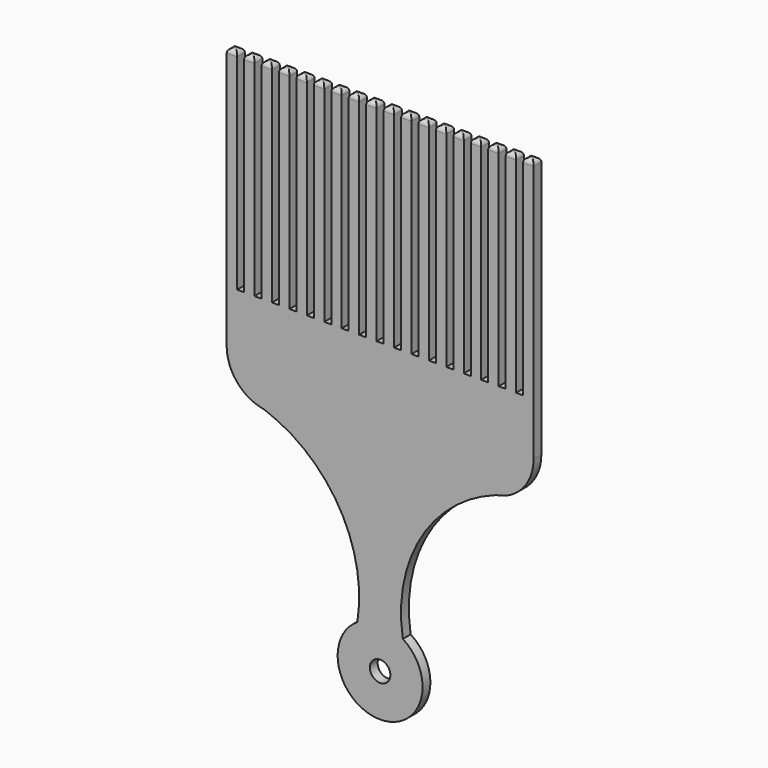
from build123d import *

# Parameters (mm, degrees)
F0_R     = 3.7382012242
F1_DEPTH = 3.556
F3_SCALE = 0.8
F4_R     = 1.27


with BuildPart() as f1:
    # F0 (on Front) → F1 (new body)
    with BuildSketch(Plane.XZ):
        with BuildLine():
            Line((-52.07, 181.6023319495), (-55.88, 181.6023319495))
            Line((-55.88, 181.6023319495), (-55.88, 86.1316665151))
            ThreePointArc((-55.88, 86.1316665151), (-52.0040063032, 75.6508869522), (-42.2413344101, 70.2139480257))
            ThreePointArc((-42.2413344101, 70.2139480257), (-14.9072200491, 47.7917837992), (-8.2826688201, 13.0639480257))
            ThreePointArc((-8.2826688201, 13.0639480257), (-14.8550807048, -4.3122984655), (0, -15.4683334849))
            ThreePointArc((0, -15.4683334849), (14.8550807048, -4.3122984655), (8.2826688201, 13.0639480257))
            ThreePointArc((8.2826688201, 13.0639480257), (14.9072200491, 47.7917837992), (42.2413344101, 70.2139480257))
            ThreePointArc((42.2413344101, 70.2139480257), (52.0040063032, 75.6508869522), (55.88, 86.1316665151))
            Line((55.88, 86.1316665151), (55.88, 181.6023319495))
            Line((55.88, 181.6023319495), (52.07, 181.6023319495))
            Line((52.07, 181.6023319495), (52.07, 105.4023319495))
            Line((52.07, 105.4023319495), (49.53, 105.4023319495))
            Line((49.53, 105.4023319495), (49.53, 181.6023319495))
            Line((49.53, 181.6023319495), (45.72, 181.6023319495))
            Line((45.72, 181.6023319495), (45.72, 105.4023319495))
            Line((45.72, 105.4023319495), (43.18, 105.4023319495))
            Line((43.18, 105.4023319495), (43.18, 181.6023319495))
            Line((43.18, 181.6023319495), (39.37, 181.6023319495))
            Line((39.37, 181.6023319495), (39.37, 105.4023319495))
            Line((39.37, 105.4023319495), (36.83, 105.4023319495))
            Line((36.83, 105.4023319495), (36.83, 181.6023319495))
            Line((36.83, 181.6023319495), (33.02, 181.6023319495))
            Line((33.02, 181.6023319495), (33.02, 105.4023319495))
            Line((33.02, 105.4023319495), (30.48, 105.4023319495))
            Line((30.48, 105.4023319495), (30.48, 181.6023319495))
            Line((30.48, 181.6023319495), (26.67, 181.6023319495))
            Line((26.67, 181.6023319495), (26.67, 105.4023319495))
            Line((26.67, 105.4023319495), (24.13, 105.4023319495))
            Line((24.13, 105.4023319495), (24.13, 181.6023319495))
            Line((24.13, 181.6023319495), (20.32, 181.6023319495))
            Line((20.32, 181.6023319495), (20.32, 105.4023319495))
            Line((20.32, 105.4023319495), (17.78, 105.4023319495))
            Line((17.78, 105.4023319495), (17.78, 181.6023319495))
            Line((17.78, 181.6023319495), (13.97, 181.6023319495))
            Line((13.97, 181.6023319495), (13.97, 105.4023319495))
            Line((13.97, 105.4023319495), (11.43, 105.4023319495))
            Line((11.43, 105.4023319495), (11.43, 181.6023319495))
            Line((11.43, 181.6023319495), (7.62, 181.6023319495))
            Line((7.62, 181.6023319495), (7.62, 105.4023319495))
            Line((7.62, 105.4023319495), (5.08, 105.4023319495))
            Line((5.08, 105.4023319495), (5.08, 181.6023319495))
            Line((5.08, 181.6023319495), (1.27, 181.6023319495))
            Line((1.27, 181.6023319495), (1.27, 105.4023319495))
            Line((1.27, 105.4023319495), (-1.27, 105.4023319495))
            Line((-1.27, 105.4023319495), (-1.27, 181.6023319495))
            Line((-1.27, 181.6023319495), (-5.08, 181.6023319495))
            Line((-5.08, 181.6023319495), (-5.08, 105.4023319495))
            Line((-5.08, 105.4023319495), (-7.62, 105.4023319495))
            Line((-7.62, 105.4023319495), (-7.62, 181.6023319495))
            Line((-7.62, 181.6023319495), (-11.43, 181.6023319495))
            Line((-11.43, 181.6023319495), (-11.43, 105.4023319495))
            Line((-11.43, 105.4023319495), (-13.97, 105.4023319495))
            Line((-13.97, 105.4023319495), (-13.97, 181.6023319495))
            Line((-13.97, 181.6023319495), (-17.78, 181.6023319495))
            Line((-17.78, 181.6023319495), (-17.78, 105.4023319495))
            Line((-17.78, 105.4023319495), (-20.32, 105.4023319495))
            Line((-20.32, 105.4023319495), (-20.32, 181.6023319495))
            Line((-20.32, 181.6023319495), (-24.13, 181.6023319495))
            Line((-24.13, 181.6023319495), (-24.13, 105.4023319495))
            Line((-24.13, 105.4023319495), (-26.67, 105.4023319495))
            Line((-26.67, 105.4023319495), (-26.67, 181.6023319495))
            Line((-26.67, 181.6023319495), (-30.48, 181.6023319495))
            Line((-30.48, 181.6023319495), (-30.48, 105.4023319495))
            Line((-30.48, 105.4023319495), (-33.02, 105.4023319495))
            Line((-33.02, 105.4023319495), (-33.02, 181.6023319495))
            Line((-33.02, 181.6023319495), (-36.83, 181.6023319495))
            Line((-36.83, 181.6023319495), (-36.83, 105.4023319495))
            Line((-36.83, 105.4023319495), (-39.37, 105.4023319495))
            Line((-39.37, 105.4023319495), (-39.37, 181.6023319495))
            Line((-39.37, 181.6023319495), (-43.18, 181.6023319495))
            Line((-43.18, 181.6023319495), (-43.18, 105.4023319495))
            Line((-43.18, 105.4023319495), (-45.72, 105.4023319495))
            Line((-45.72, 105.4023319495), (-45.72, 181.6023319495))
            Line((-45.72, 181.6023319495), (-49.53, 181.6023319495))
            Line((-49.53, 181.6023319495), (-49.53, 105.4023319495))
            Line((-49.53, 105.4023319495), (-52.07, 105.4023319495))
            Line((-52.07, 105.4023319495), (-52.07, 181.6023319495))
        make_face()
        Circle(F0_R, mode=Mode.SUBTRACT)
    extrude(amount=F1_DEPTH)


with BuildPart() as f1_1:
    # F3: moved
    add(f1.part.scale(F3_SCALE))

    # F4
    f4_edges = [f1_1.edges().sort_by_distance(p)[0] for p in [
        (33.02, 0, 145.281866),
        (31.496, -1.4224, 145.281866),
        (34.544, -1.4224, 145.281866),
        (39.624, -1.4224, 145.281866),
        (36.576, -1.4224, 145.281866),
        (38.1, 0, 145.281866),
        (38.1, -2.8448, 145.281866),
        (44.704, -1.4224, 145.281866),
        (41.656, -1.4224, 145.281866),
        (43.18, 0, 145.281866),
        (43.18, -2.8448, 145.281866),
        (29.464, -1.4224, 145.281866),
        (26.416, -1.4224, 145.281866),
        (27.94, 0, 145.281866),
        (27.94, -2.8448, 145.281866),
        (24.384, -1.4224, 145.281866),
        (21.336, -1.4224, 145.281866),
        (22.86, 0, 145.281866),
        (22.86, -2.8448, 145.281866),
        (19.304, -1.4224, 145.281866),
        (16.256, -1.4224, 145.281866),
        (17.78, 0, 145.281866),
        (17.78, -2.8448, 145.281866),
        (14.224, -1.4224, 145.281866),
        (11.176, -1.4224, 145.281866),
        (12.7, 0, 145.281866),
        (12.7, -2.8448, 145.281866),
        (9.144, -1.4224, 145.281866),
        (6.096, -1.4224, 145.281866),
        (7.62, 0, 145.281866),
        (7.62, -2.8448, 145.281866),
        (4.064, -1.4224, 145.281866),
        (1.016, -1.4224, 145.281866),
        (2.54, 0, 145.281866),
        (2.54, -2.8448, 145.281866),
        (-1.016, -1.4224, 145.281866),
        (-4.064, -1.4224, 145.281866),
        (-2.54, 0, 145.281866),
        (-2.54, -2.8448, 145.281866),
        (-6.096, -1.4224, 145.281866),
        (-9.144, -1.4224, 145.281866),
        (-7.62, 0, 145.281866),
        (-7.62, -2.8448, 145.281866),
        (-11.176, -1.4224, 145.281866),
        (-14.224, -1.4224, 145.281866),
        (-12.7, 0, 145.281866),
        (-12.7, -2.8448, 145.281866),
        (-16.256, -1.4224, 145.281866),
        (-19.304, -1.4224, 145.281866),
        (-17.78, 0, 145.281866),
        (-17.78, -2.8448, 145.281866),
        (-21.336, -1.4224, 145.281866),
        (-24.384, -1.4224, 145.281866),
        (-22.86, 0, 145.281866),
        (-22.86, -2.8448, 145.281866),
        (-26.416, -1.4224, 145.281866),
        (-29.464, -1.4224, 145.281866),
        (-27.94, 0, 145.281866),
        (-27.94, -2.8448, 145.281866),
        (-31.496, -1.4224, 145.281866),
        (-34.544, -1.4224, 145.281866),
        (-33.02, 0, 145.281866),
        (-33.02, -2.8448, 145.281866),
        (-36.576, -1.4224, 145.281866),
        (-39.624, -1.4224, 145.281866),
        (-38.1, 0, 145.281866),
        (-38.1, -2.8448, 145.281866),
        (-41.656, -1.4224, 145.281866),
        (-44.704, -1.4224, 145.281866),
        (-43.18, 0, 145.281866),
        (-43.18, -2.8448, 145.281866),
        (33.02, -2.8448, 145.281866),
    ]]
    fillet(f4_edges, radius=F4_R)


solid = f1_1.part
